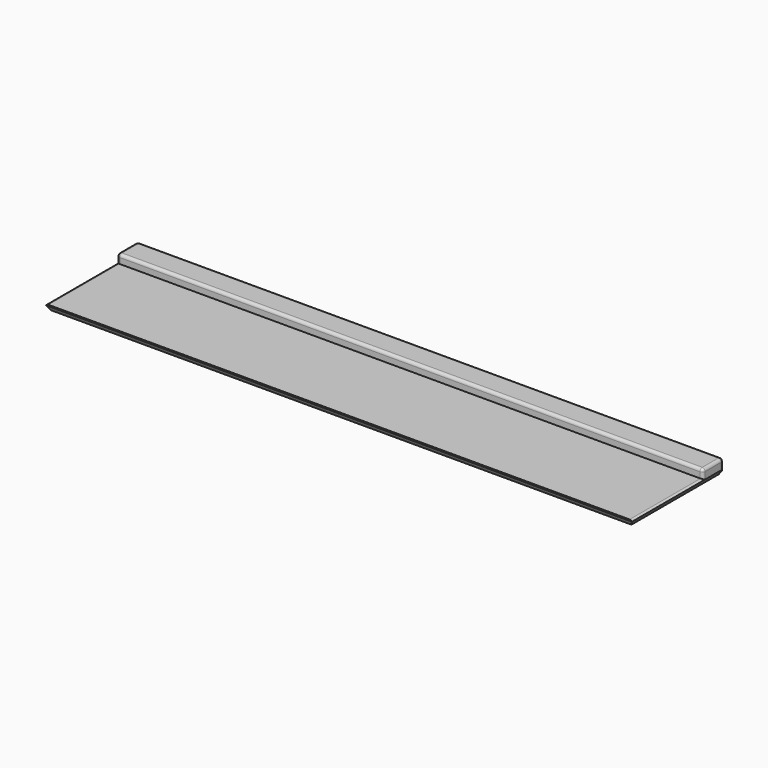
from build123d import *

# Parameters (mm, degrees)
F0_W         = 102.5
F0_H         = 20
F1_DEPTH     = 1
F2_W         = 102.5
F2_H         = 4.5
F3_DEPTH     = 1.5
F4_C1_SIZE2  = 0.45
F4_C1_SIZE   = 0.7794228634
F4_C2_SIZE2  = 0.7794228634
F4_C2_SIZE   = 0.45
F4_C3_SIZE2  = 0.7794228634
F4_C3_SIZE   = 0.45
F4_C4_SIZE2  = 0.7794228634
F4_C4_SIZE   = 0.45
F5_T1_DEPTH  = 2.4705771366
F5_T3_DEPTH  = 1
F5_T5_DEPTH  = 3.5
F5_T7_DEPTH  = 101.5
F5_T9_DEPTH  = 16.5365895505
F5_S13_W     = 0.51
F5_S13_H     = 0.51
F5_T14_DEPTH = 0.51
F5_S19_W     = 0.51
F5_S19_H     = 0.51
F5_T20_DEPTH = 0.51
F5_S25_W     = 0.51
F5_S25_H     = 0.51
F5_T26_DEPTH = 0.51
F5_S31_W     = 0.51
F5_S31_H     = 0.51
F5_T32_DEPTH = 0.51
F5_T39_DEPTH = 16.5365895505
F5_T43_DEPTH = 2.25
F5_T52_DEPTH = 16.5365895505
F5_T56_DEPTH = 2.25


# Not quite as in the source:
# - a fillet or chamfer that OpenCascade refuses, or shapes differently, is made with other operations: its cross-section is extruded or revolved along the edge and cut away or added


with BuildPart() as f1:
    # F0 (on Top) → F1 (new body)
    with BuildSketch(Plane.XY):
        with Locations((-51.25, 10)):
            Rectangle(F0_W, F0_H)
    extrude(amount=F1_DEPTH)

    # F2 (on face) → F3 (join)
    with BuildSketch(Plane.XY.offset(1)):
        with Locations((-51.25, 17.75)):
            Rectangle(F2_W, F2_H)
    extrude(amount=F3_DEPTH)

    # F4: chamfer of 0.45 x 0.7794228634 on 4 edges, made by hand

    # F4_c1
    f4_c1_edges = [f1.edges().sort_by_distance(p)[0] for p in [
        (-51.25, 0, 0),
    ]]
    f4_c1_side = f1.faces().sort_by_distance((-51.25, 0, 0.009))[0]
    chamfer(f4_c1_edges, length=F4_C1_SIZE, length2=F4_C1_SIZE2, reference=f4_c1_side)

    # F4_c2
    f4_c2_edges = [f1.edges().sort_by_distance(p)[0] for p in [
        (-51.25, 20, 0),
    ]]
    f4_c2_side = f1.faces().sort_by_distance((-51.25, 19.991, 0))[0]
    chamfer(f4_c2_edges, length=F4_C2_SIZE, length2=F4_C2_SIZE2, reference=f4_c2_side)

    # F4_c3
    f4_c3_edges = [f1.edges().sort_by_distance(p)[0] for p in [
        (0, 10, 0),
    ]]
    f4_c3_side = f1.faces().sort_by_distance((-0.009, 10, 0))[0]
    chamfer(f4_c3_edges, length=F4_C3_SIZE, length2=F4_C3_SIZE2, reference=f4_c3_side)

    # F4_c4
    f4_c4_edges = [f1.edges().sort_by_distance(p)[0] for p in [
        (-102.5, 10, 0),
    ]]
    f4_c4_side = f1.faces().sort_by_distance((-102.491, 10, 0))[0]
    chamfer(f4_c4_edges, length=F4_C4_SIZE, length2=F4_C4_SIZE2, reference=f4_c4_side)

    # F5: fillet of radius 0.5 on 10 edges, made by hand

    # F5_s2 → F5_t1 (cut)
    with BuildSketch(Plane.XY.offset(-0.4705771366)):
        with BuildLine():
            ThreePointArc((-102, 20), (-102.3535533906, 19.8535533906), (-102.5, 19.5))
            Line((-102.5, 19.5), (-102.5, 20))
            Line((-102.5, 20), (-102, 20))
        make_face()
        with BuildLine():
            ThreePointArc((-0.5, 20), (-0.1464466094, 19.8535533906), (0, 19.5))
            Line((0, 19.5), (0, 20))
            Line((0, 20), (-0.5, 20))
        make_face()
    extrude(amount=F5_T1_DEPTH, mode=Mode.SUBTRACT)

    # F5_s4 → F5_t3 (cut)
    with BuildSketch(Plane.XY.offset(1)):
        with BuildLine():
            ThreePointArc((-102.5, 16), (-102.3535533906, 15.6464466094), (-102, 15.5))
            Line((-102, 15.5), (-102.5, 15.5))
            Line((-102.5, 15.5), (-102.5, 16))
        make_face()
        with BuildLine():
            ThreePointArc((0, 16), (-0.1464466094, 15.6464466094), (-0.5, 15.5))
            Line((-0.5, 15.5), (0, 15.5))
            Line((0, 15.5), (0, 16))
        make_face()
    extrude(amount=F5_T3_DEPTH, mode=Mode.SUBTRACT)

    # F5_s6 → F5_t5 (cut)
    with BuildSketch(Plane.XZ.offset(-19.5)):
        with BuildLine():
            ThreePointArc((-102.5, 2), (-102.3535533906, 2.3535533906), (-102, 2.5))
            Line((-102, 2.5), (-102.5, 2.5))
            Line((-102.5, 2.5), (-102.5, 2))
        make_face()
        with BuildLine():
            ThreePointArc((0, 2), (-0.1464466094, 2.3535533906), (-0.5, 2.5))
            Line((-0.5, 2.5), (0, 2.5))
            Line((0, 2.5), (0, 2))
        make_face()
    extrude(amount=F5_T5_DEPTH, mode=Mode.SUBTRACT)

    # F5_s8 → F5_t7 (cut)
    with BuildSketch(Plane.YZ.offset(-102)):
        with BuildLine():
            ThreePointArc((20, 2), (19.8535533906, 2.3535533906), (19.5, 2.5))
            Line((19.5, 2.5), (20, 2.5))
            Line((20, 2.5), (20, 2))
        make_face()
        with BuildLine():
            ThreePointArc((16, 2.5), (15.6464466094, 2.3535533906), (15.5, 2))
            Line((15.5, 2), (15.5, 2.5))
            Line((15.5, 2.5), (16, 2.5))
        make_face()
    extrude(amount=F5_T7_DEPTH, mode=Mode.SUBTRACT)

    # F5_s10 → F5_t9 (cut)
    with BuildSketch(Plane.XZ.offset(-15.5)):
        with BuildLine():
            ThreePointArc((-102.5, 0.7794228634), (-102.3201923811, 0.9414246435), (-102.0853641798, 1))
            Line((-102.0853641798, 1), (-102.5, 1))
            Line((-102.5, 1), (-102.5, 0.7794228634))
        make_face()
        with BuildLine():
            ThreePointArc((0, 0.7794228634), (-0.1798076189, 0.9414246435), (-0.4146358202, 1))
            Line((-0.4146358202, 1), (0, 1))
            Line((0, 1), (0, 0.7794228634))
        make_face()
    extrude(amount=F5_T9_DEPTH, mode=Mode.SUBTRACT)


with BuildPart() as f5_tool12:
    # F5_s13 → F5_t14 (new body)
    with BuildSketch(Plane.XY.offset(2)):
        with Locations((-102.255, 19.755)):
            Rectangle(F5_S13_W, F5_S13_H)
    extrude(amount=F5_T14_DEPTH)

    # F5_s15 → F5_t16 (revolve, cut)
    with BuildSketch(Plane(origin=(-102, 19.5, 2), x_dir=(0.7071067812, -0.7071067812, 0), z_dir=(-0.7071067812, -0.7071067812, 0))):
        with BuildLine():
            ThreePointArc((0, -0.5), (0.5, 0), (0, 0.5))
            Line((0, 0.5), (0, -0.5))
        make_face()
    revolve(axis=Axis((-102, 19.5, 2), (0, 0, 1)), mode=Mode.SUBTRACT)


with BuildPart() as f1_1:
    add(f1.part)

    # F5_t11: cut F5_tool12
    add(f5_tool12.part, mode=Mode.SUBTRACT)


with BuildPart() as f5_tool18:
    # F5_s19 → F5_t20 (new body)
    with BuildSketch(Plane.XY.offset(2)):
        with Locations((-102.255, 15.745)):
            Rectangle(F5_S19_W, F5_S19_H)
    extrude(amount=F5_T20_DEPTH)

    # F5_s21 → F5_t22 (revolve, cut)
    with BuildSketch(Plane(origin=(-102, 16, 2), x_dir=(0.7071067812, 0.7071067812, 0), z_dir=(0.7071067812, -0.7071067812, 0))):
        with BuildLine():
            ThreePointArc((0, -0.5), (0.5, 0), (0, 0.5))
            Line((0, 0.5), (0, -0.5))
        make_face()
    revolve(axis=Axis((-102, 16, 2), (0, 0, 1)), mode=Mode.SUBTRACT)


with BuildPart() as f1_2:
    add(f1_1.part)

    # F5_t17: cut F5_tool18
    add(f5_tool18.part, mode=Mode.SUBTRACT)


with BuildPart() as f5_tool24:
    # F5_s25 → F5_t26 (new body)
    with BuildSketch(Plane.XY.offset(2)):
        with Locations((-0.245, 19.755)):
            Rectangle(F5_S25_W, F5_S25_H)
    extrude(amount=F5_T26_DEPTH)

    # F5_s27 → F5_t28 (revolve, cut)
    with BuildSketch(Plane(origin=(-0.5, 19.5, 2), x_dir=(-0.7071067812, -0.7071067812, 0), z_dir=(-0.7071067812, 0.7071067812, 0))):
        with BuildLine():
            ThreePointArc((0, -0.5), (0.5, 0), (0, 0.5))
            Line((0, 0.5), (0, -0.5))
        make_face()
    revolve(axis=Axis((-0.5, 19.5, 2), (0, 0, 1)), mode=Mode.SUBTRACT)


with BuildPart() as f1_3:
    add(f1_2.part)

    # F5_t23: cut F5_tool24
    add(f5_tool24.part, mode=Mode.SUBTRACT)


with BuildPart() as f5_tool30:
    # F5_s31 → F5_t32 (new body)
    with BuildSketch(Plane.XY.offset(2)):
        with Locations((-0.245, 15.745)):
            Rectangle(F5_S31_W, F5_S31_H)
    extrude(amount=F5_T32_DEPTH)

    # F5_s33 → F5_t34 (revolve, cut)
    with BuildSketch(Plane(origin=(-0.5, 16, 2), x_dir=(-0.7071067812, 0.7071067812, 0), z_dir=(0.7071067812, 0.7071067812, 0))):
        with BuildLine():
            ThreePointArc((0, -0.5), (0.5, 0), (0, 0.5))
            Line((0, 0.5), (0, -0.5))
        make_face()
    revolve(axis=Axis((-0.5, 16, 2), (0, 0, 1)), mode=Mode.SUBTRACT)


with BuildPart() as f1_4:
    add(f1_3.part)

    # F5_t29: cut F5_tool30
    add(f5_tool30.part, mode=Mode.SUBTRACT)


with BuildPart() as f5_tool37:
    # F5_s38 → F5_t39 (new body)
    with BuildSketch(Plane.XZ.offset(-16.5365895505)):
        with BuildLine():
            ThreePointArc((-102.5, 0.7794228634), (-102.3201923811, 0.9414246435), (-102.0853641798, 1))
            Line((-102.0853641798, 1), (-102.5, 1))
            Line((-102.5, 1), (-102.5, 0.7794228634))
        make_face()
    extrude(amount=F5_T39_DEPTH)

    split(bisect_by=Plane.XZ.offset(-15.5), keep=Keep.BOTTOM)


with BuildPart() as f5_tool41:
    # F5_s42 → F5_t43 (new body)
    with BuildSketch(Plane.XY.offset(-0.25)):
        with BuildLine():
            ThreePointArc((-102.5, 16), (-102.3535533906, 15.6464466094), (-102, 15.5))
            Line((-102, 15.5), (-102.5, 15.5))
            Line((-102.5, 15.5), (-102.5, 16))
        make_face()
    extrude(amount=F5_T43_DEPTH)

    split(bisect_by=Plane.XY, keep=Keep.TOP)

    split(bisect_by=Plane(origin=(-76.5375, 0, -44.1889462281), x_dir=(0, 1, 0), z_dir=(0.8660254038, 0, 0.5)), keep=Keep.TOP)

    split(bisect_by=Plane.XY.offset(1), keep=Keep.BOTTOM)


with BuildPart() as f5_tool37_1:
    add(f5_tool37.part)

    # F5_t47: intersect F5_tool41
    add(f5_tool41.part, mode=Mode.INTERSECT)


with BuildPart() as f1_5:
    add(f1_4.part)

    # F5_t35: cut F5_tool37
    add(f5_tool37_1.part, mode=Mode.SUBTRACT)


with BuildPart() as f5_tool50:
    # F5_s51 → F5_t52 (new body)
    with BuildSketch(Plane.XZ):
        with BuildLine():
            ThreePointArc((0, 0.7794228634), (-0.1798076189, 0.9414246435), (-0.4146358202, 1))
            Line((-0.4146358202, 1), (0, 1))
            Line((0, 1), (0, 0.7794228634))
        make_face()
    extrude(amount=-F5_T52_DEPTH)

    split(bisect_by=Plane.XZ.offset(-15.5), keep=Keep.BOTTOM)


with BuildPart() as f5_tool54:
    # F5_s55 → F5_t56 (new body)
    with BuildSketch(Plane.XY.offset(-0.25)):
        with BuildLine():
            ThreePointArc((0, 16), (-0.1464466094, 15.6464466094), (-0.5, 15.5))
            Line((-0.5, 15.5), (0, 15.5))
            Line((0, 15.5), (0, 16))
        make_face()
    extrude(amount=F5_T56_DEPTH)

    split(bisect_by=Plane.XY, keep=Keep.TOP)

    split(bisect_by=Plane(origin=(-0.3375, 0, 0.1948557159), x_dir=(0, 1, 0), z_dir=(-0.8660254038, 0, 0.5)), keep=Keep.TOP)

    split(bisect_by=Plane.XY.offset(1), keep=Keep.BOTTOM)


with BuildPart() as f5_tool50_1:
    add(f5_tool50.part)

    # F5_t60: intersect F5_tool54
    add(f5_tool54.part, mode=Mode.INTERSECT)


with BuildPart() as f1_6:
    add(f1_5.part)

    # F5_t48: cut F5_tool50
    add(f5_tool50_1.part, mode=Mode.SUBTRACT)


solid = f1_6.part
